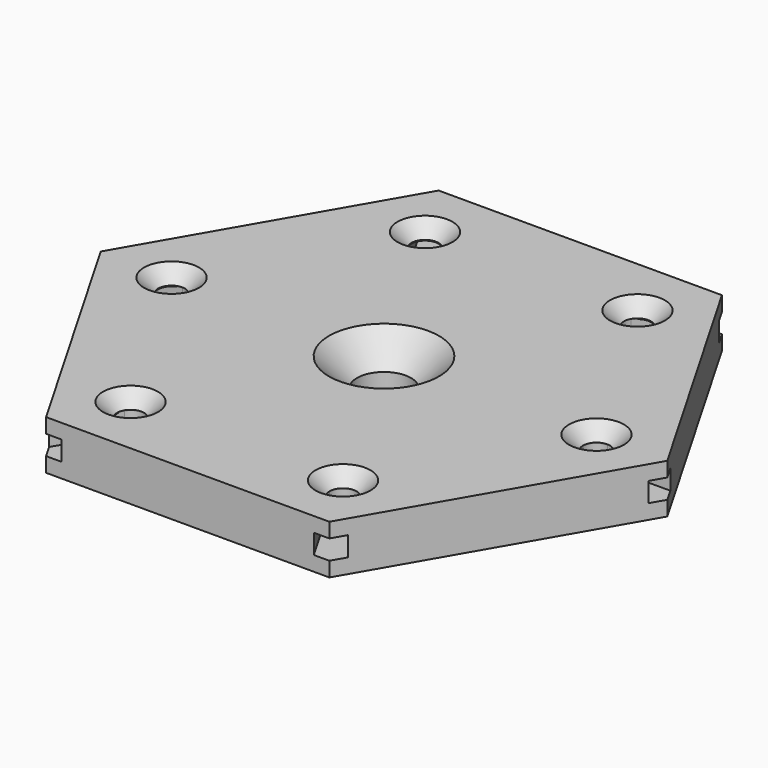
from build123d import *

# Parameters (mm, degrees)
F1_DEPTH        = 5
F4_D            = 11
F4_DEPTH        = 57.15
F4_CSINK_D      = 22.4
F4_CSINK_ANGLE  = 90
F4_TIP          = 3.3047334047
F5_D            = 5.5
F5_DEPTH        = 57.15
F5_CSINK_D      = 11.2
F5_CSINK_ANGLE  = 90
F5_TIP          = 1.6523667023
F7_DEPTH        = 2
F7_COPIES_COUNT = 6


# Not quite as in the source:
# - a pattern or mirror of a feature is missing from the dataset's text; its kind, count and spacing are read off the source's solid


with BuildPart() as f1:
    # F0 (on Top) → F1 (new body, symmetric)
    with BuildSketch(Plane.XY):
        Polygon((28.8675134595, 50), (-28.8675134595, 50), (-57.735026919, 0), (-28.8675134595, -50), (28.8675134595, -50), (57.735026919, 0), align=None)
    extrude(amount=F1_DEPTH, both=True)

    # F4
    with Locations(Plane.XY.offset(5)):
        with Locations((0, 0)):
            CounterSinkHole(F4_D / 2, F4_CSINK_D / 2, depth=F4_DEPTH, counter_sink_angle=F4_CSINK_ANGLE)
            with Locations((0, 0, -(F4_DEPTH + F4_TIP / 2))):  # 118° drill point
                Cone(0, F4_D / 2, F4_TIP, mode=Mode.SUBTRACT)

    # F5
    with Locations(Plane.XY.offset(5)):
        with Locations((21.6506350946, 37.5), (43.3012701892, 0), (21.6506350946, -37.5), (-21.6506350946, -37.5), (-43.3012701892, 0), (-21.6506350946, 37.5)):
            CounterSinkHole(F5_D / 2, F5_CSINK_D / 2, depth=F5_DEPTH, counter_sink_angle=F5_CSINK_ANGLE)
            with Locations((0, 0, -(F5_DEPTH + F5_TIP / 2))):  # 118° drill point
                Cone(0, F5_D / 2, F5_TIP, mode=Mode.SUBTRACT)

    # F6 (on Top) → F7 (cut, symmetric)
    with BuildSketch(Plane.XY):
        with BuildLine():
            ThreePointArc((-19.2690652342, -38.875), (-18.9943390723, -38.211752374), (-18.9006350946, -37.5))
            ThreePointArc((-18.9006350946, -37.5), (-20.9388827206, -34.8437039777), (-24.032204955, -36.125))
            ThreePointArc((-24.032204955, -36.125), (-23.0256350946, -39.8815698604), (-19.2690652342, -38.875))
        make_face()
        with BuildLine():
            ThreePointArc((-19.2690652342, -38.875), (-23.0256350946, -39.8815698604), (-24.032204955, -36.125))
            Line((-24.032204955, -36.125), (-30.4552266998, -47.25))
            Line((-30.4552266998, -47.25), (-28.8675134595, -50))
            Line((-28.8675134595, -50), (-25.6920869789, -50))
            Line((-25.6920869789, -50), (-19.2690652342, -38.875))
        make_face()
    f7 = extrude(amount=F7_DEPTH, both=True, mode=Mode.SUBTRACT)

    # F7_copies: F7 ×6 about axis
    f7_copies_axis = Axis((0, 0, 0), (0, 0, 1))
    for i in range(1, F7_COPIES_COUNT):
        add(f7.rotate(f7_copies_axis, i * 360 / F7_COPIES_COUNT), mode=Mode.SUBTRACT)


solid = f1.part
